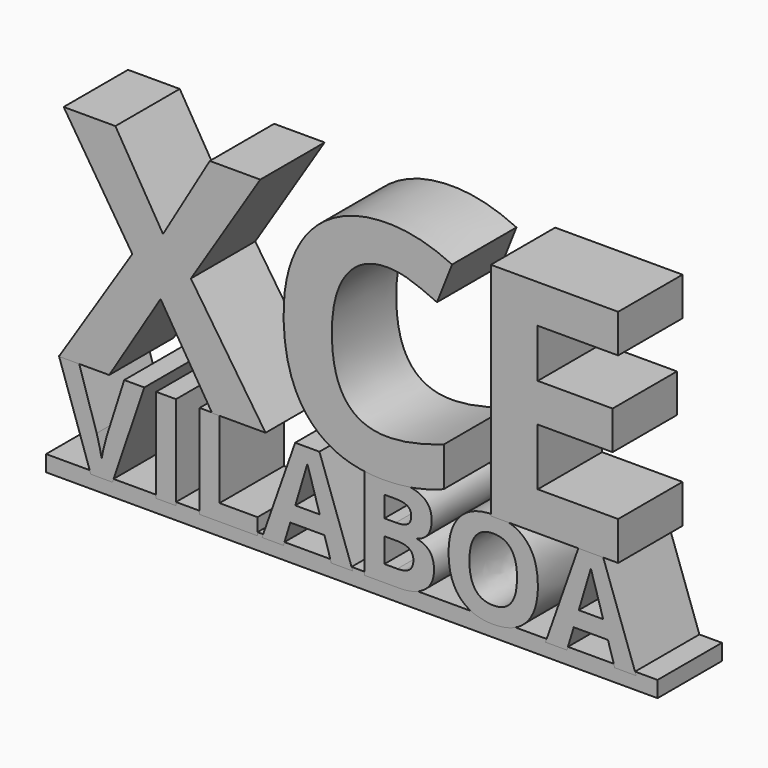
from build123d import *

# Parameters (mm, degrees)
F0_W         = 190
F0_H         = 25
F1_DEPTH     = 5
F2_TEXT_SIZE = 40.8200455581
F3_DEPTH     = 25
F4_TEXT_SIZE = 96.256684492
F5_DEPTH     = 25


# Not quite as in the source:
# - Text() gives the source's letters only with a copy of the font that has no kerning and outlines rounded to 1/6400 em; it was checked with that copy


with BuildPart() as f1:
    # F0 (on Top) → F1 (new body)
    with BuildSketch(Plane.XY):
        with Locations((0, -25.1305297149)):
            Rectangle(F0_W, F0_H)
    extrude(amount=F1_DEPTH)


with BuildPart() as f3:
    # F2 (on face) → F3 (new body)
    with BuildSketch(Plane.XZ.offset(37.6305297149)):
        with Locations((-91, 4)):
            Text('VILABOA', F2_TEXT_SIZE, font='Open Sans', font_style=FontStyle.BOLD, text_align=(TextAlign.LEFT, TextAlign.BOTTOM))
    extrude(amount=-F3_DEPTH)


with BuildPart() as f5:
    # F4 (on face) → F5 (new body)
    with BuildSketch(Plane.XZ.offset(37.6305297149)):
        with Locations((-91, 33)):
            Text('XCE', F4_TEXT_SIZE, font='Open Sans', font_style=FontStyle.BOLD, text_align=(TextAlign.LEFT, TextAlign.BOTTOM))
    extrude(amount=-F5_DEPTH)


solid = Compound([f1.part, f3.part, f5.part])
